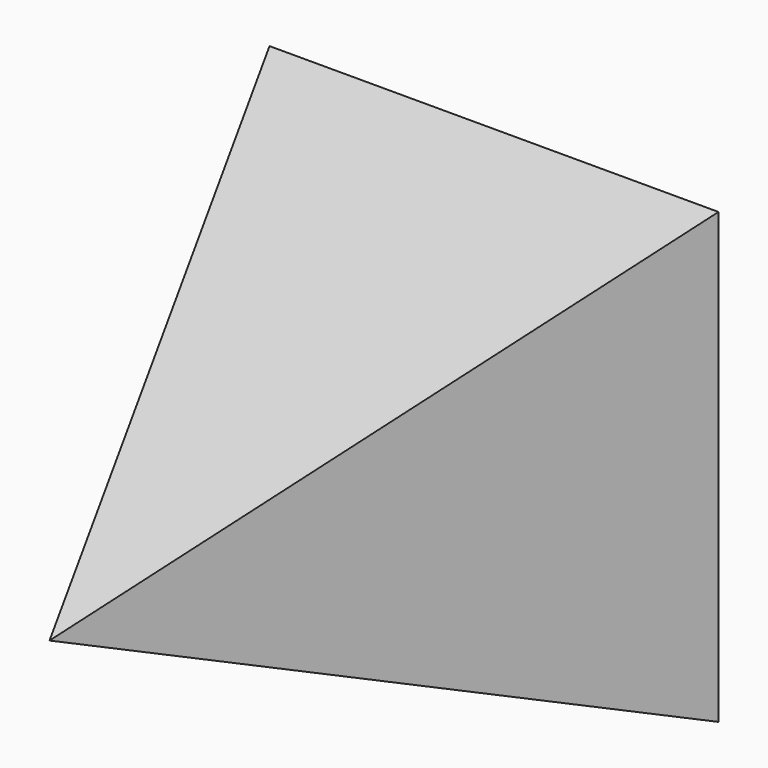
from build123d import *

# Parameters (mm, degrees)
F0_W      = 50.8
F0_H      = 50.8
F1_FACE_W = 50.8
F1_FACE_H = 50.8


# Not quite as in the source:
# - an extrude whose draft closes it to a point is written as a loft to that point


with BuildPart() as f1:
    # F0 (on Front) → F1 section 0
    with BuildSketch(Plane.XZ, mode=Mode.PRIVATE) as f1_s0:
        Rectangle(F0_W, F0_H)
    loft([f1_s0.sketch, Vertex(0, -62.8672060768, 0)], ruled=True)

    # F1_face (on face) → F2 section 0
    with BuildSketch(Plane(origin=(0, 0, 0), x_dir=(1, 0, 0), z_dir=(0, 1, 0)), mode=Mode.PRIVATE) as f2_s0:
        Rectangle(F1_FACE_W, F1_FACE_H)
    loft([f2_s0.sketch, Vertex(0, 14.6646968374, 0)], ruled=True)


solid = f1.part
